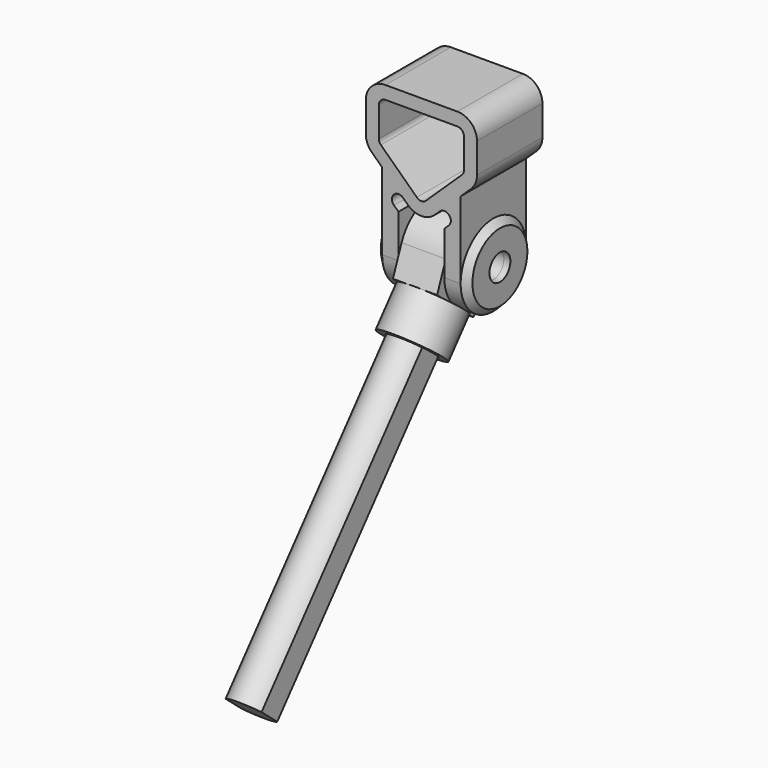
from build123d import *

# Parameters (mm, degrees)
F1_DEPTH  = 25
F3_DEPTH  = 25
F2_R      = 12.5
F2_R_2    = 4
F4_DEPTH  = 2
F5_SIZE   = 1.99999
F6_R      = 12.5
F7_DEPTH  = 2
F8_SIZE   = 1.99999
F9_DEPTH  = 30
F10_R     = 4
F11_DEPTH = 6.75
F13_DEPTH = 108
F12_R     = 9.5
F12_R_2   = 7
F14_DEPTH = 12.5


# Not quite as in the source:
# - a fillet or chamfer is up to 0.001 mm smaller than in the source, because OpenCascade refuses the exact size


with BuildPart() as f1:
    # F0 (on Front) → F1 (new body)
    with BuildSketch(Plane.XZ):
        with BuildLine():
            ThreePointArc((-17, 30.8538616003), (-16.5181427671, 28.4979964934), (-15.1499665327, 26.520528267))
            Line((-15.1499665327, 26.520528267), (-12, 23.5038538771))
            Line((-12, 23.5038538771), (-12, -12.5))
            Line((-12, -12.5), (-7, -12.5))
            Line((-7, -12.5), (-7, 13.1769694163))
            Line((-7, 13.1769694163), (-8.3833221776, 14.5017557411))
            ThreePointArc((-8.3833221776, 14.5017557411), (-8.4444444444, 17.3295223631), (-5.6166778224, 17.39064463))
            Line((-5.6166778224, 17.39064463), (-4.1499665327, 15.9859978379))
            ThreePointArc((-4.1499665327, 15.9859978379), (0, 14.3193311712), (4.1499665327, 15.9859978379))
            Line((4.1499665327, 15.9859978379), (5.6166778224, 17.39064463))
            ThreePointArc((5.6166778224, 17.39064463), (8.4444444444, 17.3295223631), (8.3833221776, 14.5017557411))
            Line((8.3833221776, 14.5017557411), (7, 13.1769694163))
            Line((7, 13.1769694163), (7, -12.5))
            Line((7, -12.5), (12, -12.5))
            Line((12, -12.5), (12, 23.5038538771))
            Line((12, 23.5038538771), (15.1499665327, 26.520528267))
            ThreePointArc((15.1499665327, 26.520528267), (16.5181427671, 28.4979964934), (17, 30.8538616003))
            Line((17, 30.8538616003), (17, 40))
            ThreePointArc((17, 40), (15.2426406871, 44.2426406871), (11, 46))
            Line((11, 46), (0, 46))
            Line((0, 46), (-11, 46))
            ThreePointArc((-11, 46), (-15.2426406871, 44.2426406871), (-17, 40))
            Line((-17, 40), (-17, 30.8538616003))
        make_face()
        with BuildLine():
            Line((-11, 42), (0, 42))
            Line((0, 42), (11, 42))
            ThreePointArc((11, 42), (12.4142135624, 41.4142135624), (13, 40))
            Line((13, 40), (13, 30.8538616003))
            ThreePointArc((13, 30.8538616003), (12.8393809224, 30.0685732313), (12.3833221776, 29.4094171559))
            Line((12.3833221776, 29.4094171559), (1.3833221776, 18.8748867268))
            ThreePointArc((1.3833221776, 18.8748867268), (0, 18.3193311712), (-1.3833221776, 18.8748867268))
            Line((-1.3833221776, 18.8748867268), (-12.3833221776, 29.4094171559))
            ThreePointArc((-12.3833221776, 29.4094171559), (-12.8393809224, 30.0685732313), (-13, 30.8538616003))
            Line((-13, 30.8538616003), (-13, 40))
            ThreePointArc((-13, 40), (-12.4142135624, 41.4142135624), (-11, 42))
        make_face(mode=Mode.SUBTRACT)
    extrude(amount=F1_DEPTH)

    # F2 (on face) → F3 (cut)
    with BuildSketch(Plane.YZ.offset(12)):
        with BuildLine():
            ThreePointArc((-12.5, -12.5), (-21.3388347734, -8.8388347563), (-25, 2.41e-08))
            Line((-25, 2.41e-08), (-25, -12.5))
            Line((-25, -12.5), (-12.5, -12.5))
        make_face()
        with BuildLine():
            Line((0, -12.5), (0, 0))
            ThreePointArc((0, 0), (-3.6611652352, -8.8388347648), (-12.5, -12.5))
            Line((-12.5, -12.5), (0, -12.5))
        make_face()
    extrude(amount=-F3_DEPTH, mode=Mode.SUBTRACT)

    # F2 (on face) → F4 (join)
    with BuildSketch(Plane.YZ.offset(12)):
        with Locations((-12.5, 0)):
            Circle(F2_R)
        with Locations((-12.5, 0)):
            Circle(F2_R_2, mode=Mode.SUBTRACT)
    extrude(amount=F4_DEPTH)

    # F5 (size 2 in the source; OpenCascade refuses exactly that, so slightly less here)
    f5_edges = [f1.edges().sort_by_distance(p)[0] for p in [
        (14, -25, 0),
    ]]
    chamfer(f5_edges, length=F5_SIZE)

    # F6 (on face) → F7 (join)
    with BuildSketch(Plane(origin=(-12, 0, 0), x_dir=(0, -1, 0), z_dir=(-1, 0, 0))):
        with Locations((12.5, 0)):
            Circle(F6_R)
    extrude(amount=F7_DEPTH)

    # F8 (size 2 in the source; OpenCascade refuses exactly that, so slightly less here)
    f8_edges = [f1.edges().sort_by_distance(p)[0] for p in [
        (-14, 0, 0),
    ]]
    chamfer(f8_edges, length=F8_SIZE)

    # F2 (on face) → F9 (cut)
    with BuildSketch(Plane.YZ.offset(12)):
        with Locations((-12.5, 0)):
            Circle(F2_R_2)
    extrude(amount=-F9_DEPTH, mode=Mode.SUBTRACT)


with BuildPart() as f11:
    # F10 (on Right) → F11 (new body, symmetric)
    with BuildSketch(Plane.YZ):
        with BuildLine():
            Line((-13.640445133, -15.3606440262), (-5.9673218086, -10.6571157284))
            ThreePointArc((-5.9673218086, -10.6571157284), (-4.4651548789, 9.575555539), (-24.1295978573, 4.5828434054))
            Line((-24.1295978573, 4.5828434054), (-27.4292451092, -3.7904670518))
            Line((-27.4292451092, -3.7904670518), (-20.5348451211, -9.575555539))
            Line((-20.5348451211, -9.575555539), (-13.640445133, -15.3606440262))
        make_face()
        with Locations((-12.5, 0)):
            Circle(F10_R, mode=Mode.SUBTRACT)
    extrude(amount=F11_DEPTH, both=True)

    # F12 (on face) → F13 (join)
    with BuildSketch(Plane(origin=(0, -13.1995440107, -15.7306039953), x_dir=(1, 0, 0), z_dir=(0, -0.6427876097, -0.7660444431))):
        with BuildLine():
            Line((5.5, 5.6624365784), (5.5, 13.4886744996))
            ThreePointArc((5.5, 13.4886744996), (0, 16.325555539), (-5.5, 13.4886744996))
            Line((-5.5, 13.4886744996), (-5.5, 5.6624365784))
            ThreePointArc((-5.5, 5.6624365784), (0, 2.825555539), (5.5, 5.6624365784))
        make_face()
    extrude(amount=F13_DEPTH)


with BuildPart() as f14:
    # F12 (on face) → F14 (new body)
    with BuildSketch(Plane(origin=(0, -13.1995440107, -15.7306039953), x_dir=(1, 0, 0), z_dir=(0, -0.6427876097, -0.7660444431))):
        with Locations((0, 9.575555539)):
            Circle(F12_R)
        with Locations((0, 9.575555539)):
            Circle(F12_R_2, mode=Mode.SUBTRACT)
    extrude(amount=F14_DEPTH)


solid = Compound([f1.part, f11.part, f14.part])
